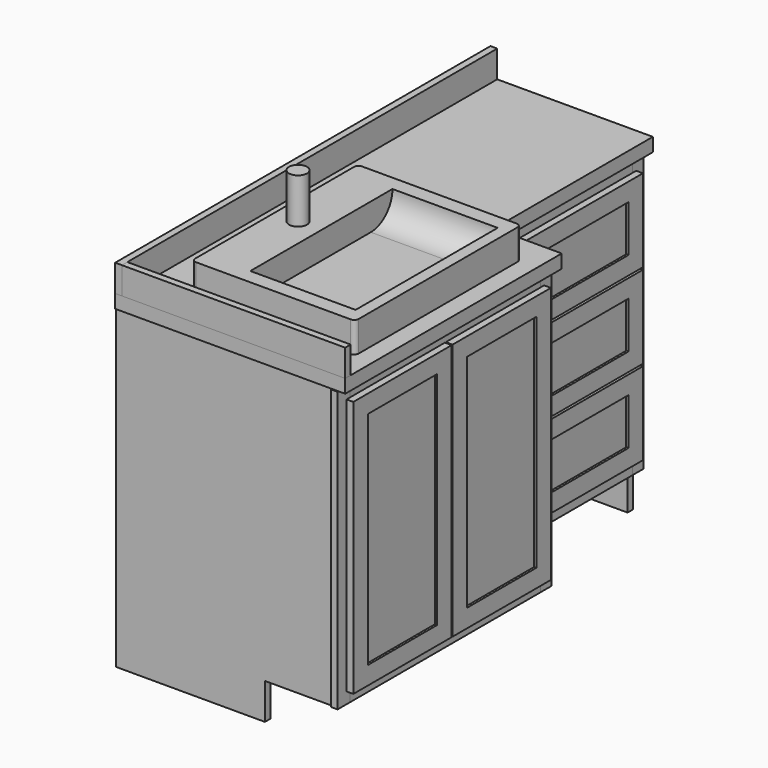
from build123d import *

# Parameters (mm, degrees)
F1_W      = 609.6
F1_H      = 19.05
F2_DEPTH  = 889
F1_W_2    = 419.1
F3_W      = 190.5
F3_H      = 101.6
F4_DEPTH  = 1295.401
F5_W      = 44.45
F5_H      = 787.4
F6_DEPTH  = 19.05
F5_W_2    = 38.1
F7_W      = 38.1
F7_H      = 787.4
F8_DEPTH  = 19.05
F10_DEPTH = 19.05
F11_W     = 419.1
F11_H     = 19.05
F12_DEPTH = 120.65
F13_W     = 19.05
F13_H     = 768.35
F14_DEPTH = 19.05
F15_W     = 669.925
F15_H     = 44.45
F16_DEPTH = 19.05
F17_W     = 19.05
F17_H     = 50.8
F18_DEPTH = 492.125
F19_W     = 19.05
F19_H     = 88.9
F20_DEPTH = 1257.3
F21_W     = 88.9
F21_H     = 19.05
F22_DEPTH = 701.675
F23_W     = 88.9
F23_H     = 19.05
F24_DEPTH = 536.575
F26_DEPTH = 19.05
F27_W     = 346.075
F27_H     = 723.9
F28_DEPTH = 19.05
F29_W     = 244.475
F29_H     = 622.3
F30_DEPTH = 6.35
F31_W     = 517.525
F31_H     = 232.8333333333
F32_DEPTH = 19.05
F33_W     = 415.925
F33_H     = 131.2333333333
F34_DEPTH = 6.35
F36_DEPTH = 38.1
F37_W     = 19.05
F37_H     = 1320.8
F38_DEPTH = 76.2
F39_W     = 628.65
F39_H     = 19.05
F40_DEPTH = 76.2
F42_DEPTH = 85.725
F43_W     = 296.2960004807
F43_H     = 500.0777393579
F44_DEPTH = 76.2
F45_R     = 76.19999
F46_R     = 25.3021956534
F47_DEPTH = 127
F48_W     = 19.05
F48_H     = 88.9
F49_DEPTH = 1257.3


# Not quite as in the source:
# - a fillet or chamfer is up to 0.001 mm smaller than in the source, because OpenCascade refuses the exact size


with BuildPart() as f2:
    # F1 (on Top) → F2 (new body)
    with BuildSketch(Plane.XY):
        with Locations((-942.975, 12.7)):
            Rectangle(F1_W, F1_H)
    extrude(amount=F2_DEPTH)


with BuildPart() as f2b:
    # F1 (on Top) → F2, piece 2 (new body)
    with BuildSketch(Plane.XY):
        with Locations((-942.975, 733.425)):
            Rectangle(F1_W, F1_H)
    extrude(amount=F2_DEPTH)


with BuildPart() as f2c:
    # F1 (on Top) → F2, piece 3 (new body)
    with BuildSketch(Plane.XY):
        with Locations((-1038.225, 1289.05)):
            Rectangle(F1_W_2, F1_H)
    extrude(amount=F2_DEPTH)


with BuildPart() as f4_tool:
    # F3 (on face) → F4 (new body, through all)
    with BuildSketch(Plane.XZ.offset(-3.175)):
        with Locations((-733.425, 50.8)):
            Rectangle(F3_W, F3_H)
    extrude(amount=-F4_DEPTH)


with BuildPart() as f2_1:
    add(f2.part)

    # F4: cut by f4_tool
    add(f4_tool.part, mode=Mode.SUBTRACT)


with BuildPart() as f2b_1:
    add(f2b.part)

    # F4: cut by f4_tool
    add(f4_tool.part, mode=Mode.SUBTRACT)

    # F11 (on face) → F12 (cut)
    with BuildSketch(Plane(origin=(0, 0, 0), x_dir=(1, 0, 0), z_dir=(0, 0, -1))):
        with Locations((-1038.225, -733.425)):
            Rectangle(F11_W, F11_H)
    extrude(amount=-F12_DEPTH, mode=Mode.SUBTRACT)

    # F13 (on face) → F14 (cut, through all)
    with BuildSketch(Plane(origin=(0, 742.95, 0), x_dir=(-1, 0, 0), z_dir=(0, 1, 0))):
        with Locations((1238.25, 504.825)):
            Rectangle(F13_W, F13_H)
    extrude(amount=-F14_DEPTH, mode=Mode.SUBTRACT)


with BuildPart() as f6:
    # F5 (on face) → F6 (new body)
    with BuildSketch(Plane.YZ.offset(-638.175)):
        with Locations((19.05, 495.3)):
            Rectangle(F5_W, F5_H)
    extrude(amount=F6_DEPTH)


with BuildPart() as f6b:
    # F5 (on face) → F6, piece 2 (new body)
    with BuildSketch(Plane.YZ.offset(-638.175)):
        with Locations((730.25, 495.3)):
            Rectangle(F5_W_2, F5_H)
    extrude(amount=F6_DEPTH)


with BuildPart() as f8:
    # F7 (on face) → F8 (new body)
    with BuildSketch(Plane.YZ.offset(-828.675)):
        with Locations((1292.225, 495.3)):
            Rectangle(F7_W, F7_H)
    extrude(amount=F8_DEPTH)


with BuildPart() as f8b:
    # F7 (on face) → F8, piece 2 (new body)
    with BuildSketch(Plane.YZ.offset(-828.675)):
        with Locations((762, 495.3)):
            Rectangle(F7_W, F7_H)
    extrude(amount=F8_DEPTH)


with BuildPart() as f10:
    # F9 (on face) → F10 (new body)
    with BuildSketch(Plane(origin=(0, 0, 101.6), x_dir=(1, 0, 0), z_dir=(0, 0, -1))):
        Polygon((-638.175, -723.9), (-638.175, -22.225), (-1228.725, -22.225), (-1228.725, -1279.525), (-828.675, -1279.525), (-828.675, -723.9), align=None)
    extrude(amount=-F10_DEPTH)


with BuildPart() as f16:
    # F15 (on face) → F16 (new body)
    with BuildSketch(Plane.YZ.offset(-619.125)):
        with Locations((376.2375, 866.775)):
            Rectangle(F15_W, F15_H)
    extrude(amount=-F16_DEPTH)


with BuildPart() as f16b:
    # F15 (on face) → F16, piece 2 (new body)
    with BuildSketch(Plane.YZ.offset(-619.125)):
        with Locations((376.2375, 123.825)):
            Rectangle(F15_W, F15_H)
    extrude(amount=-F16_DEPTH)


with BuildPart() as f18:
    # F17 (on face) → F18 (new body, through all)
    with BuildSketch(Plane(origin=(0, 781.05, 0), x_dir=(-1, 0, 0), z_dir=(0, 1, 0))):
        with Locations((819.15, 863.6)):
            Rectangle(F17_W, F17_H)
    extrude(amount=F18_DEPTH)


with BuildPart() as f18b:
    # F17 (on face) → F18, piece 2 (new body, through all)
    with BuildSketch(Plane(origin=(0, 781.05, 0), x_dir=(-1, 0, 0), z_dir=(0, 1, 0))):
        with Locations((819.15, 127)):
            Rectangle(F17_W, F17_H)
    extrude(amount=F18_DEPTH)


with BuildPart() as f20:
    # F19 (on face) → F20 (new body, through all)
    with BuildSketch(Plane(origin=(0, 22.225, 0), x_dir=(-1, 0, 0), z_dir=(0, 1, 0))):
        with Locations((1238.25, 844.55)):
            Rectangle(F19_W, F19_H)
    extrude(amount=F20_DEPTH)


with BuildPart() as f20b:
    # F19 (on face) → F20, piece 2 (new body, through all)
    with BuildSketch(Plane(origin=(0, 22.225, 0), x_dir=(-1, 0, 0), z_dir=(0, 1, 0))):
        with Locations((1238.25, 146.05)):
            Rectangle(F19_W, F19_H)
    extrude(amount=F20_DEPTH)


with BuildPart() as f22:
    # F21 (on face) → F22 (new body, through all)
    with BuildSketch(Plane(origin=(0, 22.225, 0), x_dir=(-1, 0, 0), z_dir=(0, 1, 0))):
        with Locations((682.625, 879.475)):
            Rectangle(F21_W, F21_H)
    extrude(amount=F22_DEPTH)


with BuildPart() as f24:
    # F23 (on face) → F24 (new body, through all)
    with BuildSketch(Plane(origin=(0, 742.95, 0), x_dir=(-1, 0, 0), z_dir=(0, 1, 0))):
        with Locations((873.125, 879.475)):
            Rectangle(F23_W, F23_H)
    extrude(amount=F24_DEPTH)


with BuildPart() as f26:
    # F25 (on face) → F26 (new body)
    with BuildSketch(Plane.XY.offset(889)):
        Polygon((-1228.725, 22.225), (-1152.525, 22.225), (-1228.725, 98.425), align=None)
    extrude(amount=-F26_DEPTH)


with BuildPart() as f26b:
    # F25 (on face) → F26, piece 2 (new body)
    with BuildSketch(Plane.XY.offset(889)):
        Polygon((-1228.725, 723.9), (-1228.725, 647.7), (-1152.525, 723.9), align=None)
    extrude(amount=-F26_DEPTH)


with BuildPart() as f26c:
    # F25 (on face) → F26, piece 3 (new body)
    with BuildSketch(Plane.XY.offset(889)):
        Polygon((-1228.725, 742.95), (-1152.525, 742.95), (-1228.725, 819.15), align=None)
    extrude(amount=-F26_DEPTH)


with BuildPart() as f26d:
    # F25 (on face) → F26, piece 4 (new body)
    with BuildSketch(Plane.XY.offset(889)):
        Polygon((-1228.725, 1279.525), (-1228.725, 1203.325), (-1152.525, 1279.525), align=None)
    extrude(amount=-F26_DEPTH)


with BuildPart() as f28:
    # F27 (on face) → F28 (new body)
    with BuildSketch(Plane.YZ.offset(-619.125)):
        with Locations((201.6125, 495.3)):
            Rectangle(F27_W, F27_H)
    extrude(amount=F28_DEPTH)


with BuildPart() as f28b:
    # F27 (on face) → F28, piece 2 (new body)
    with BuildSketch(Plane.YZ.offset(-619.125)):
        with Locations((550.8625, 495.3)):
            Rectangle(F27_W, F27_H)
    extrude(amount=F28_DEPTH)


with BuildPart() as f30_tool:
    # F29 (on face) → F30 (new body)
    with BuildSketch(Plane.YZ.offset(-600.075)):
        with Locations((201.6125, 495.3)):
            Rectangle(F29_W, F29_H)
        with Locations((550.8625, 495.3)):
            Rectangle(F29_W, F29_H)
    extrude(amount=-F30_DEPTH)


with BuildPart() as f28_1:
    add(f28.part)

    # F30: cut by f30_tool
    add(f30_tool.part, mode=Mode.SUBTRACT)


with BuildPart() as f28b_1:
    add(f28b.part)

    # F30: cut by f30_tool
    add(f30_tool.part, mode=Mode.SUBTRACT)


with BuildPart() as f32:
    # F31 (on face) → F32 (new body)
    with BuildSketch(Plane.YZ.offset(-809.625)):
        with Locations((1027.1125, 734.4833333333)):
            Rectangle(F31_W, F31_H)
    extrude(amount=F32_DEPTH)


with BuildPart() as f32b:
    # F31 (on face) → F32, piece 2 (new body)
    with BuildSketch(Plane.YZ.offset(-809.625)):
        with Locations((1027.1125, 495.3)):
            Rectangle(F31_W, F31_H)
    extrude(amount=F32_DEPTH)


with BuildPart() as f32c:
    # F31 (on face) → F32, piece 3 (new body)
    with BuildSketch(Plane.YZ.offset(-809.625)):
        with Locations((1027.1125, 256.1166666667)):
            Rectangle(F31_W, F31_H)
    extrude(amount=F32_DEPTH)


with BuildPart() as f34_tool:
    # F33 (on face) → F34 (new body)
    with BuildSketch(Plane.YZ.offset(-790.575)):
        with Locations((1027.1125, 734.4833333333)):
            Rectangle(F33_W, F33_H)
        with Locations((1027.1125, 495.3)):
            Rectangle(F33_W, F33_H)
        with Locations((1027.1125, 256.1166666667)):
            Rectangle(F33_W, F33_H)
    extrude(amount=-F34_DEPTH)


with BuildPart() as f32_1:
    add(f32.part)

    # F34: cut by f34_tool
    add(f34_tool.part, mode=Mode.SUBTRACT)


with BuildPart() as f32b_1:
    add(f32b.part)

    # F34: cut by f34_tool
    add(f34_tool.part, mode=Mode.SUBTRACT)


with BuildPart() as f32c_1:
    add(f32c.part)

    # F34: cut by f34_tool
    add(f34_tool.part, mode=Mode.SUBTRACT)


with BuildPart() as f36:
    # F35 (on face) → F36 (new body)
    with BuildSketch(Plane.XY.offset(889)):
        Polygon((-790.575, 1320.8), (-1247.775, 1320.8), (-1247.775, 0), (-600.075, 0), (-600.075, 762), (-790.575, 762), align=None)
    extrude(amount=F36_DEPTH)


with BuildPart() as f38:
    # F37 (on face) → F38 (new body)
    with BuildSketch(Plane.XY.offset(927.1)):
        with Locations((-1238.25, 660.4)):
            Rectangle(F37_W, F37_H)
    extrude(amount=F38_DEPTH)


with BuildPart() as f40:
    # F39 (on face) → F40 (new body)
    with BuildSketch(Plane.XY.offset(927.1)):
        with Locations((-914.4, 9.525)):
            Rectangle(F39_W, F39_H)
    extrude(amount=F40_DEPTH)


with BuildPart() as f42:
    # F41 (on face) → F42 (new body)
    with BuildSketch(Plane.XY.offset(927.1)):
        with BuildLine():
            ThreePointArc((-650.875, 669.925), (-654.5947438789, 678.9052561211), (-663.575, 682.625))
            Line((-663.575, 682.625), (-1098.55, 682.625))
            ThreePointArc((-1098.55, 682.625), (-1107.5302561211, 678.9052561211), (-1111.25, 669.925))
            Line((-1111.25, 669.925), (-1111.25, 111.125))
            ThreePointArc((-1111.25, 111.125), (-1107.5302561211, 102.1447438789), (-1098.55, 98.425))
            Line((-1098.55, 98.425), (-663.575, 98.425))
            ThreePointArc((-663.575, 98.425), (-654.5947438789, 102.1447438789), (-650.875, 111.125))
            Line((-650.875, 111.125), (-650.875, 669.925))
        make_face()
    extrude(amount=F42_DEPTH)

    # F43 (on face) → F44 (cut)
    with BuildSketch(Plane.XY.offset(1012.825)):
        with Locations((-831.3964605331, 390.525)):
            Rectangle(F43_W, F43_H)
    extrude(amount=-F44_DEPTH, mode=Mode.SUBTRACT)

    # F45 (radius 76.2 in the source; OpenCascade refuses exactly that, so slightly less here)
    f45_edges = [f42.edges().sort_by_distance(p)[0] for p in [
        (-831.396461, 640.56387, 936.625),
        (-831.396461, 140.48613, 936.625),
        (-683.24846, 390.525, 936.625),
    ]]
    fillet(f45_edges, radius=F45_R)


with BuildPart() as f47:
    # F46 (on face) → F47 (new body)
    with BuildSketch(Plane.XY.offset(1012.825)):
        with Locations((-1045.3972303867, 390.525)):
            Circle(F46_R)
    extrude(amount=F47_DEPTH)


with BuildPart() as f49:
    # F48 (on face) → F49 (new body, through all)
    with BuildSketch(Plane(origin=(0, 22.225, 0), x_dir=(-1, 0, 0), z_dir=(0, 1, 0))):
        with Locations((1238.25, 844.55)):
            Rectangle(F48_W, F48_H)
    extrude(amount=F49_DEPTH)


solid = Compound([f2c.part, f2_1.part, f2b_1.part, f6.part, f6b.part, f8.part, f8b.part, f10.part, f16.part, f16b.part, f18.part, f18b.part, f20.part, f20b.part, f22.part, f24.part, f26.part, f26b.part, f26c.part, f26d.part, f28_1.part, f28b_1.part, f32_1.part, f32b_1.part, f32c_1.part, f36.part, f38.part, f40.part, f42.part, f47.part, f49.part])
